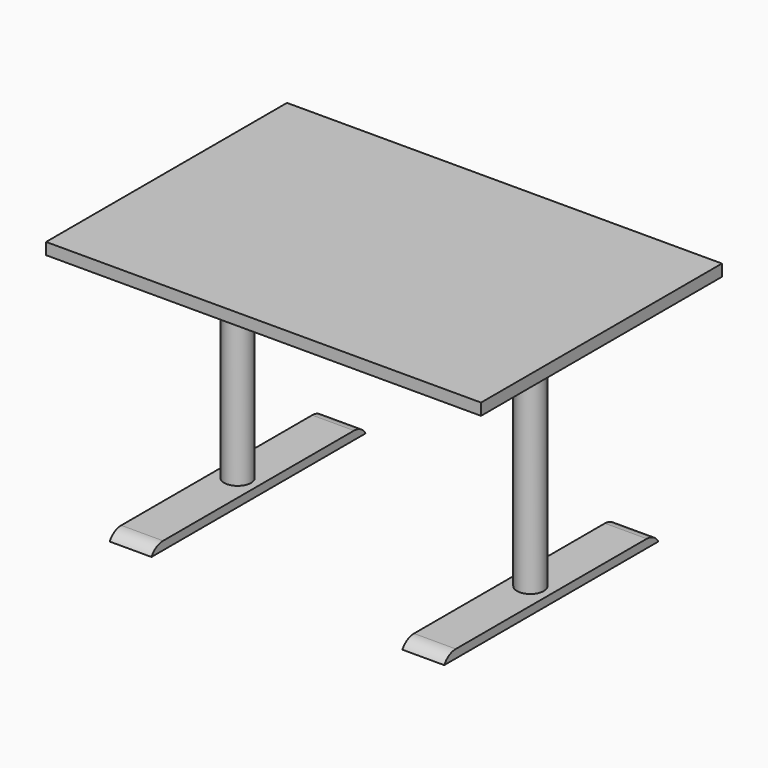
from build123d import *

# Parameters (mm, degrees)
F0_W        = 1300
F0_H        = 900
F1_DEPTH    = 35
F2_W        = 125
F2_H        = 500
F3_DEPTH    = 75
F4_R        = 40
F5_R        = 40
F6_DEPTH    = 625
F7_W        = 125
F7_H        = 800
F7_R        = 40
F8_DEPTH    = 25
F9_T1_DEPTH = 341.5063509461
F9_T3_DEPTH = 341.5063509461


# Not quite as in the source:
# - a fillet or chamfer that OpenCascade refuses, or shapes differently, is made with other operations: its cross-section is extruded or revolved along the edge and cut away or added


with BuildPart() as f1:
    # F0 (on Top) → F1 (new body)
    with BuildSketch(Plane.XY):
        with Locations((-10.7608698308, 73.6055876629)):
            Rectangle(F0_W, F0_H)
    extrude(amount=F1_DEPTH)

    # F2 (on face) → F3 (join)
    with BuildSketch(Plane(origin=(0, 0, 0), x_dir=(1, 0, 0), z_dir=(0, 0, -1))):
        with Locations((-448.2608698308, -73.6055876629)):
            Rectangle(F2_W, F2_H)
        with Locations((426.7391301692, -73.6055876629)):
            Rectangle(F2_W, F2_H)
    extrude(amount=F3_DEPTH)

    # F4 (on face) + F5 (on face) → F6 (join)
    with BuildSketch(Plane(origin=(0, 0, -75), x_dir=(1, 0, 0), z_dir=(0, 0, -1))):
        with Locations((-448.2608698308, -73.6055876629)):
            Circle(F4_R)
    with BuildSketch(Plane(origin=(0, 0, -75), x_dir=(1, 0, 0), z_dir=(0, 0, -1))):
        with Locations((426.7391301692, -73.6055876629)):
            Circle(F5_R)
    extrude(amount=F6_DEPTH)

    # F7 (on face) → F8 (join)
    with BuildSketch(Plane(origin=(0, 0, -700), x_dir=(1, 0, 0), z_dir=(0, 0, -1))):
        with Locations((-448.2608698308, -73.6055876629)):
            Rectangle(F7_W, F7_H)
        with Locations((-448.2608698308, -73.6055876629)):
            Circle(F7_R, mode=Mode.SUBTRACT)
        with Locations((426.7391301692, -73.6055876629)):
            Rectangle(F7_W, F7_H)
        with Locations((-448.2608698308, -73.6055876629)):
            Circle(F7_R)
    extrude(amount=F8_DEPTH)

    # F9: fillet of radius 50 on 4 edges, made by hand

    # F9_s2 → F9_t1 (cut)
    with BuildSketch(Plane.YZ.offset(-619.0140453039)):
        with BuildLine():
            ThreePointArc((-283.0931421479, -700), (-308.0931421479, -706.6987298108), (-326.3944123371, -725))
            Line((-326.3944123371, -725), (-326.3944123371, -700))
            Line((-326.3944123371, -700), (-283.0931421479, -700))
        make_face()
        with BuildLine():
            ThreePointArc((430.3043174737, -700), (455.3043174737, -706.6987298108), (473.6055876629, -725))
            Line((473.6055876629, -725), (473.6055876629, -700))
            Line((473.6055876629, -700), (430.3043174737, -700))
        make_face()
    extrude(amount=F9_T1_DEPTH, mode=Mode.SUBTRACT)

    # F9_s4 → F9_t3 (cut)
    with BuildSketch(Plane.YZ.offset(255.9859546961)):
        with BuildLine():
            ThreePointArc((-326.3944123371, -725), (-308.0931421479, -706.6987298108), (-283.0931421479, -700))
            Line((-283.0931421479, -700), (-326.3944123371, -700))
            Line((-326.3944123371, -700), (-326.3944123371, -725))
        make_face()
        with BuildLine():
            ThreePointArc((473.6055876629, -725), (455.3043174737, -706.6987298108), (430.3043174737, -700))
            Line((430.3043174737, -700), (473.6055876629, -700))
            Line((473.6055876629, -700), (473.6055876629, -725))
        make_face()
    extrude(amount=F9_T3_DEPTH, mode=Mode.SUBTRACT)


solid = f1.part
